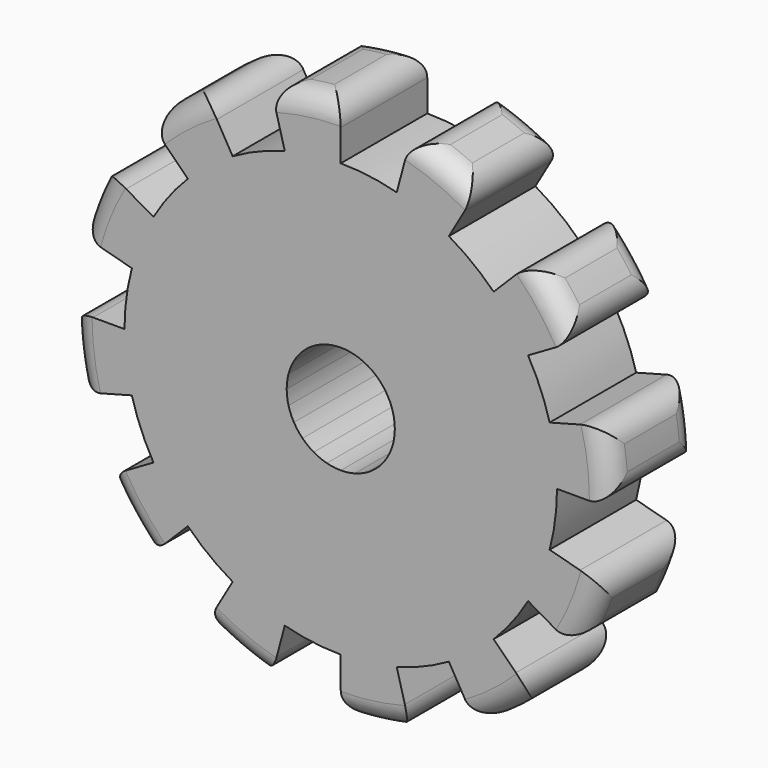
from build123d import *

# Parameters (mm, degrees)
F1_DEPTH = 25.4
F2_R     = 5.08
F3_R     = 5.08


# Not quite as in the source:
# - a feature names something its author has since deleted; it is built from what else it names


with BuildPart() as f1:
    # F0 (on Front) → F1 (new body)
    with BuildSketch(Plane.XZ):
        with BuildLine():
            Line((-61.3362899694, 16.435009364), (-49.0690319755, 13.1480074912))
            ThreePointArc((-49.0690319755, 13.1480074912), (-46.9330802516, 19.4403183641), (-43.9940905122, 25.4))
            Line((-43.9940905122, 25.4), (-54.9926131403, 31.75))
            ThreePointArc((-54.9926131403, 31.75), (-58.6663503145, 24.3003979552), (-61.3362899694, 16.435009364))
        make_face()
        with BuildLine():
            ThreePointArc((-13.1480074912, 49.0690319755), (-6.6307305648, 50.3653989578), (0, 50.8))
            Line((0, 50.8), (0, 63.5))
            ThreePointArc((0, 63.5), (-8.288413206, 62.9567486972), (-16.435009364, 61.3362899694))
            Line((-16.435009364, 61.3362899694), (-13.1480074912, 49.0690319755))
        make_face()
        with BuildLine():
            Line((13.1480074912, 49.0690319755), (3.2870018728, 12.2672579939))
            ThreePointArc((3.2870018728, 12.2672579939), (4.860079591, 11.7332700629), (6.35, 10.9985226281))
            Line((6.35, 10.9985226281), (25.4, 43.9940905122))
            ThreePointArc((25.4, 43.9940905122), (19.4403183641, 46.9330802516), (13.1480074912, 49.0690319755))
        make_face()
        with BuildLine():
            ThreePointArc((43.9940905122, -25.4), (46.9330802516, -19.4403183641), (49.0690319755, -13.1480074912))
            Line((49.0690319755, -13.1480074912), (12.2672579939, -3.2870018728))
            ThreePointArc((12.2672579939, -3.2870018728), (11.7332700629, -4.860079591), (10.9985226281, -6.35))
            Line((10.9985226281, -6.35), (43.9940905122, -25.4))
        make_face()
        with BuildLine():
            ThreePointArc((25.4, -43.9940905122), (30.9250805936, -40.3023496868), (35.9210244843, -35.9210244843))
            Line((35.9210244843, -35.9210244843), (8.9802561211, -8.9802561211))
            ThreePointArc((8.9802561211, -8.9802561211), (7.7312701484, -10.0755874217), (6.35, -10.9985226281))
            Line((6.35, -10.9985226281), (25.4, -43.9940905122))
        make_face()
        with BuildLine():
            Line((13.1480074912, -49.0690319755), (3.2870018728, -12.2672579939))
            ThreePointArc((3.2870018728, -12.2672579939), (1.6576826412, -12.5913497394), (0, -12.7))
            Line((0, -12.7), (0, -50.8))
            ThreePointArc((0, -50.8), (6.6307305648, -50.3653989578), (13.1480074912, -49.0690319755))
        make_face()
        with BuildLine():
            Line((-13.1480074912, -49.0690319755), (-3.2870018728, -12.2672579939))
            ThreePointArc((-3.2870018728, -12.2672579939), (-4.860079591, -11.7332700629), (-6.35, -10.9985226281))
            Line((-6.35, -10.9985226281), (-25.4, -43.9940905122))
            ThreePointArc((-25.4, -43.9940905122), (-19.4403183641, -46.9330802516), (-13.1480074912, -49.0690319755))
        make_face()
        with BuildLine():
            Line((-35.9210244843, -35.9210244843), (-8.9802561211, -8.9802561211))
            ThreePointArc((-8.9802561211, -8.9802561211), (-10.0755874217, -7.7312701484), (-10.9985226281, -6.35))
            Line((-10.9985226281, -6.35), (-43.9940905122, -25.4))
            ThreePointArc((-43.9940905122, -25.4), (-40.3023496868, -30.9250805936), (-35.9210244843, -35.9210244843))
        make_face()
        with BuildLine():
            Line((-49.0690319755, -13.1480074912), (-12.2672579939, -3.2870018728))
            ThreePointArc((-12.2672579939, -3.2870018728), (-12.5913497394, -1.6576826412), (-12.7, 0))
            Line((-12.7, 0), (-50.8, 0))
            ThreePointArc((-50.8, 0), (-50.3653989578, -6.6307305648), (-49.0690319755, -13.1480074912))
        make_face()
        with BuildLine():
            Line((-44.9012806053, 44.9012806053), (-35.9210244843, 35.9210244843))
            ThreePointArc((-35.9210244843, 35.9210244843), (-30.9250805936, 40.3023496868), (-25.4, 43.9940905122))
            Line((-25.4, 43.9940905122), (-31.75, 54.9926131403))
            ThreePointArc((-31.75, 54.9926131403), (-38.6563507421, 50.3779371085), (-44.9012806053, 44.9012806053))
        make_face()
        with BuildLine():
            Line((25.4, 43.9940905122), (31.75, 54.9926131403))
            ThreePointArc((31.75, 54.9926131403), (24.3003979552, 58.6663503145), (16.435009364, 61.3362899694))
            Line((16.435009364, 61.3362899694), (13.1480074912, 49.0690319755))
            ThreePointArc((13.1480074912, 49.0690319755), (19.4403183641, 46.9330802516), (25.4, 43.9940905122))
        make_face()
        with BuildLine():
            Line((43.9940905122, 25.4), (54.9926131403, 31.75))
            ThreePointArc((54.9926131403, 31.75), (50.3779371085, 38.6563507421), (44.9012806053, 44.9012806053))
            Line((44.9012806053, 44.9012806053), (35.9210244843, 35.9210244843))
            ThreePointArc((35.9210244843, 35.9210244843), (40.3023496868, 30.9250805936), (43.9940905122, 25.4))
        make_face()
        with BuildLine():
            Line((50.8, 0), (63.5, 0))
            ThreePointArc((63.5, 0), (62.9567486972, 8.288413206), (61.3362899694, 16.435009364))
            Line((61.3362899694, 16.435009364), (49.0690319755, 13.1480074912))
            ThreePointArc((49.0690319755, 13.1480074912), (50.3653989578, 6.6307305648), (50.8, 0))
        make_face()
        with BuildLine():
            ThreePointArc((54.9926131403, -31.75), (58.6663503145, -24.3003979552), (61.3362899694, -16.435009364))
            Line((61.3362899694, -16.435009364), (49.0690319755, -13.1480074912))
            ThreePointArc((49.0690319755, -13.1480074912), (46.9330802516, -19.4403183641), (43.9940905122, -25.4))
            Line((43.9940905122, -25.4), (54.9926131403, -31.75))
        make_face()
        with BuildLine():
            ThreePointArc((31.75, -54.9926131403), (38.6563507421, -50.3779371085), (44.9012806053, -44.9012806053))
            Line((44.9012806053, -44.9012806053), (35.9210244843, -35.9210244843))
            ThreePointArc((35.9210244843, -35.9210244843), (30.9250805936, -40.3023496868), (25.4, -43.9940905122))
            Line((25.4, -43.9940905122), (31.75, -54.9926131403))
        make_face()
        with BuildLine():
            ThreePointArc((0, -63.5), (8.288413206, -62.9567486972), (16.435009364, -61.3362899694))
            Line((16.435009364, -61.3362899694), (13.1480074912, -49.0690319755))
            ThreePointArc((13.1480074912, -49.0690319755), (6.6307305648, -50.3653989578), (0, -50.8))
            Line((0, -50.8), (0, -63.5))
        make_face()
        with BuildLine():
            Line((-16.435009364, -61.3362899694), (-13.1480074912, -49.0690319755))
            ThreePointArc((-13.1480074912, -49.0690319755), (-19.4403183641, -46.9330802516), (-25.4, -43.9940905122))
            Line((-25.4, -43.9940905122), (-31.75, -54.9926131403))
            ThreePointArc((-31.75, -54.9926131403), (-24.3003979552, -58.6663503145), (-16.435009364, -61.3362899694))
        make_face()
        with BuildLine():
            Line((-44.9012806053, -44.9012806053), (-35.9210244843, -35.9210244843))
            ThreePointArc((-35.9210244843, -35.9210244843), (-40.3023496868, -30.9250805936), (-43.9940905122, -25.4))
            Line((-43.9940905122, -25.4), (-54.9926131403, -31.75))
            ThreePointArc((-54.9926131403, -31.75), (-50.3779371085, -38.6563507421), (-44.9012806053, -44.9012806053))
        make_face()
        with BuildLine():
            Line((-61.3362899694, -16.435009364), (-49.0690319755, -13.1480074912))
            ThreePointArc((-49.0690319755, -13.1480074912), (-50.3653989578, -6.6307305648), (-50.8, 0))
            Line((-50.8, 0), (-63.5, 0))
            ThreePointArc((-63.5, 0), (-62.9567486972, -8.288413206), (-61.3362899694, -16.435009364))
        make_face()
        with BuildLine():
            Line((-49.0690319755, 13.1480074912), (-12.2672579939, 3.2870018728))
            ThreePointArc((-12.2672579939, 3.2870018728), (-11.7332700629, 4.860079591), (-10.9985226281, 6.35))
            Line((-10.9985226281, 6.35), (-43.9940905122, 25.4))
            ThreePointArc((-43.9940905122, 25.4), (-46.9330802516, 19.4403183641), (-49.0690319755, 13.1480074912))
        make_face()
        with BuildLine():
            Line((-35.9210244843, 35.9210244843), (-8.9802561211, 8.9802561211))
            ThreePointArc((-8.9802561211, 8.9802561211), (-7.7312701484, 10.0755874217), (-6.35, 10.9985226281))
            Line((-6.35, 10.9985226281), (-25.4, 43.9940905122))
            ThreePointArc((-25.4, 43.9940905122), (-30.9250805936, 40.3023496868), (-35.9210244843, 35.9210244843))
        make_face()
        with BuildLine():
            ThreePointArc((-3.2870018728, 12.2672579939), (-1.6576826412, 12.5913497394), (0, 12.7))
            Line((0, 12.7), (0, 50.8))
            ThreePointArc((0, 50.8), (-6.6307305648, 50.3653989578), (-13.1480074912, 49.0690319755))
            Line((-13.1480074912, 49.0690319755), (-3.2870018728, 12.2672579939))
        make_face()
        with BuildLine():
            Line((10.9985226281, 6.35), (43.9940905122, 25.4))
            ThreePointArc((43.9940905122, 25.4), (40.3023496868, 30.9250805936), (35.9210244843, 35.9210244843))
            Line((35.9210244843, 35.9210244843), (8.9802561211, 8.9802561211))
            ThreePointArc((8.9802561211, 8.9802561211), (10.0755874217, 7.7312701484), (10.9985226281, 6.35))
        make_face()
        with BuildLine():
            Line((12.7, 0), (50.8, 0))
            ThreePointArc((50.8, 0), (50.3653989578, 6.6307305648), (49.0690319755, 13.1480074912))
            Line((49.0690319755, 13.1480074912), (12.2672579939, 3.2870018728))
            ThreePointArc((12.2672579939, 3.2870018728), (12.5913497394, 1.6576826412), (12.7, 0))
        make_face()
        with BuildLine():
            ThreePointArc((49.0690319755, -13.1480074912), (50.3653989578, -6.6307305648), (50.8, 0))
            Line((50.8, 0), (12.7, 0))
            ThreePointArc((12.7, 0), (12.5913497394, -1.6576826412), (12.2672579939, -3.2870018728))
            Line((12.2672579939, -3.2870018728), (49.0690319755, -13.1480074912))
        make_face()
        with BuildLine():
            ThreePointArc((35.9210244843, -35.9210244843), (40.3023496868, -30.9250805936), (43.9940905122, -25.4))
            Line((43.9940905122, -25.4), (10.9985226281, -6.35))
            ThreePointArc((10.9985226281, -6.35), (10.0755874217, -7.7312701484), (8.9802561211, -8.9802561211))
            Line((8.9802561211, -8.9802561211), (35.9210244843, -35.9210244843))
        make_face()
        with BuildLine():
            Line((25.4, -43.9940905122), (6.35, -10.9985226281))
            ThreePointArc((6.35, -10.9985226281), (4.860079591, -11.7332700629), (3.2870018728, -12.2672579939))
            Line((3.2870018728, -12.2672579939), (13.1480074912, -49.0690319755))
            ThreePointArc((13.1480074912, -49.0690319755), (19.4403183641, -46.9330802516), (25.4, -43.9940905122))
        make_face()
        with BuildLine():
            Line((0, -50.8), (0, -12.7))
            ThreePointArc((0, -12.7), (-1.6576826412, -12.5913497394), (-3.2870018728, -12.2672579939))
            Line((-3.2870018728, -12.2672579939), (-13.1480074912, -49.0690319755))
            ThreePointArc((-13.1480074912, -49.0690319755), (-6.6307305648, -50.3653989578), (0, -50.8))
        make_face()
        with BuildLine():
            Line((-25.4, -43.9940905122), (-6.35, -10.9985226281))
            ThreePointArc((-6.35, -10.9985226281), (-7.7312701484, -10.0755874217), (-8.9802561211, -8.9802561211))
            Line((-8.9802561211, -8.9802561211), (-35.9210244843, -35.9210244843))
            ThreePointArc((-35.9210244843, -35.9210244843), (-30.9250805936, -40.3023496868), (-25.4, -43.9940905122))
        make_face()
        with BuildLine():
            Line((-43.9940905122, -25.4), (-10.9985226281, -6.35))
            ThreePointArc((-10.9985226281, -6.35), (-11.7332700629, -4.860079591), (-12.2672579939, -3.2870018728))
            Line((-12.2672579939, -3.2870018728), (-49.0690319755, -13.1480074912))
            ThreePointArc((-49.0690319755, -13.1480074912), (-46.9330802516, -19.4403183641), (-43.9940905122, -25.4))
        make_face()
        with BuildLine():
            ThreePointArc((-12.7, 0), (-12.5913497394, 1.6576826412), (-12.2672579939, 3.2870018728))
            Line((-12.2672579939, 3.2870018728), (-49.0690319755, 13.1480074912))
            ThreePointArc((-49.0690319755, 13.1480074912), (-50.3653989578, 6.6307305648), (-50.8, 0))
            Line((-50.8, 0), (-12.7, 0))
        make_face()
        with BuildLine():
            Line((-43.9940905122, 25.4), (-10.9985226281, 6.35))
            ThreePointArc((-10.9985226281, 6.35), (-10.0755874217, 7.7312701484), (-8.9802561211, 8.9802561211))
            Line((-8.9802561211, 8.9802561211), (-35.9210244843, 35.9210244843))
            ThreePointArc((-35.9210244843, 35.9210244843), (-40.3023496868, 30.9250805936), (-43.9940905122, 25.4))
        make_face()
        with BuildLine():
            Line((-25.4, 43.9940905122), (-6.35, 10.9985226281))
            ThreePointArc((-6.35, 10.9985226281), (-4.860079591, 11.7332700629), (-3.2870018728, 12.2672579939))
            Line((-3.2870018728, 12.2672579939), (-13.1480074912, 49.0690319755))
            ThreePointArc((-13.1480074912, 49.0690319755), (-19.4403183641, 46.9330802516), (-25.4, 43.9940905122))
        make_face()
        with BuildLine():
            Line((0, 50.8), (0, 12.7))
            ThreePointArc((0, 12.7), (1.6576826412, 12.5913497394), (3.2870018728, 12.2672579939))
            Line((3.2870018728, 12.2672579939), (13.1480074912, 49.0690319755))
            ThreePointArc((13.1480074912, 49.0690319755), (6.6307305648, 50.3653989578), (0, 50.8))
        make_face()
        with BuildLine():
            Line((8.9802561211, 8.9802561211), (35.9210244843, 35.9210244843))
            ThreePointArc((35.9210244843, 35.9210244843), (30.9250805936, 40.3023496868), (25.4, 43.9940905122))
            Line((25.4, 43.9940905122), (6.35, 10.9985226281))
            ThreePointArc((6.35, 10.9985226281), (7.7312701484, 10.0755874217), (8.9802561211, 8.9802561211))
        make_face()
        with BuildLine():
            Line((12.2672579939, 3.2870018728), (49.0690319755, 13.1480074912))
            ThreePointArc((49.0690319755, 13.1480074912), (46.9330802516, 19.4403183641), (43.9940905122, 25.4))
            Line((43.9940905122, 25.4), (10.9985226281, 6.35))
            ThreePointArc((10.9985226281, 6.35), (11.7332700629, 4.860079591), (12.2672579939, 3.2870018728))
        make_face()
    extrude(amount=F1_DEPTH)

    # F2
    f2_edges = [f1.edges().sort_by_distance(p)[0] for p in [
        (-31.75, -12.7, 54.992613),
        (-44.901281, -12.7, 44.901281),
        (-38.656351, 0, 50.377937),
        (-38.656351, -25.4, 50.377937),
        (-54.992613, -12.7, 31.75),
        (-61.33629, -12.7, 16.435009),
        (-58.66635, 0, 24.300398),
        (-58.66635, -25.4, 24.300398),
        (-63.5, -12.7, 0),
        (-61.33629, -12.7, -16.435009),
        (-62.956749, 0, -8.288413),
        (-62.956749, -25.4, -8.288413),
    ]]
    fillet(f2_edges, radius=F2_R)

    # F3
    f3_edges = [f1.edges().sort_by_distance(p)[0] for p in [
        (0, -12.7, 63.5),
        (-16.435009, -12.7, 61.33629),
        (-8.288413, 0, 62.956749),
        (-8.288413, -25.4, 62.956749),
        (31.75, -12.7, 54.992613),
        (16.435009, -12.7, 61.33629),
        (24.300398, 0, 58.66635),
        (24.300398, -25.4, 58.66635),
        (54.992613, -12.7, 31.75),
        (44.901281, -12.7, 44.901281),
        (50.377937, 0, 38.656351),
        (50.377937, -25.4, 38.656351),
        (63.5, -12.7, 0),
        (61.33629, -12.7, 16.435009),
        (62.956749, 0, 8.288413),
        (62.956749, -25.4, 8.288413),
        (54.992613, -12.7, -31.75),
        (61.33629, -12.7, -16.435009),
        (58.66635, 0, -24.300398),
        (58.66635, -25.4, -24.300398),
        (31.75, -12.7, -54.992613),
        (44.901281, -12.7, -44.901281),
        (38.656351, 0, -50.377937),
        (38.656351, -25.4, -50.377937),
        (0, -12.7, -63.5),
        (8.288413, 0, -62.956749),
        (-31.75, -12.7, -54.992613),
        (-16.435009, -12.7, -61.33629),
        (-24.300398, 0, -58.66635),
        (-24.300398, -25.4, -58.66635),
        (-54.992613, -12.7, -31.75),
        (-44.901281, -12.7, -44.901281),
        (-50.377937, 0, -38.656351),
        (-50.377937, -25.4, -38.656351),
        (16.435009, -12.7, -61.33629),
        (8.288413, -25.4, -62.956749),
    ]]
    fillet(f3_edges, radius=F3_R)


solid = f1.part
